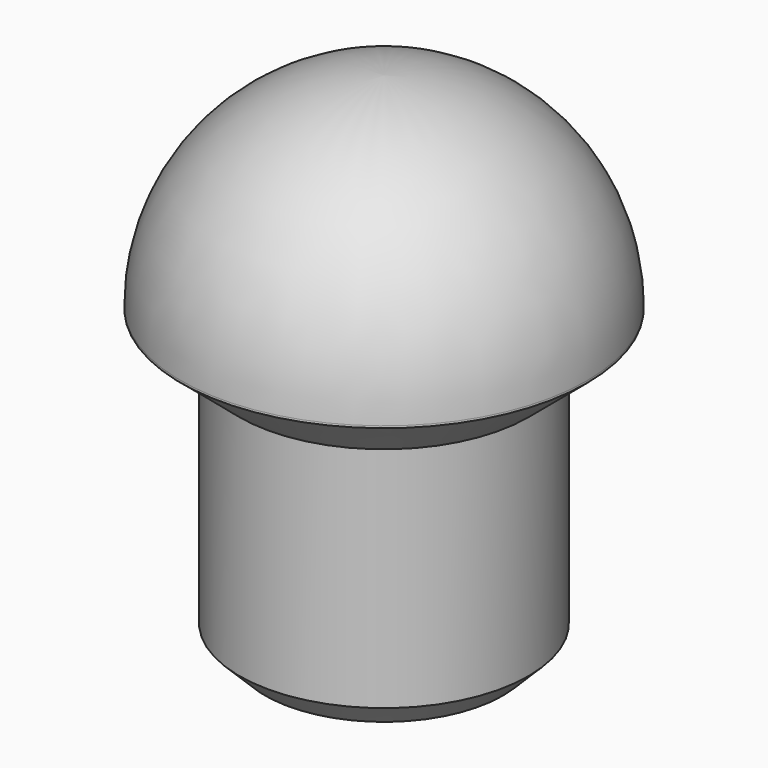
from build123d import *

# Parameters (mm, degrees)
F0_R        = 4
F0_R_2      = 2.85
F1_DEPTH    = 4
F2_DEPTH    = 6
F3_R        = 3.99999
F4_SIZE     = 0.5
F5_S5_R     = 4
F5_T6_DEPTH = 7


# Not quite as in the source:
# - a fillet or chamfer that OpenCascade refuses, or shapes differently, is made with other operations: its cross-section is extruded or revolved along the edge and cut away or added
# - a fillet or chamfer is up to 0.001 mm smaller than in the source, because OpenCascade refuses the exact size


with BuildPart() as f1:
    # F0 (on Top) → F1 (new body)
    with BuildSketch(Plane.XY):
        Circle(F0_R)
        Circle(F0_R_2, mode=Mode.SUBTRACT)
        Circle(F0_R_2)
    extrude(amount=F1_DEPTH)

    # F0 (on Top) → F2 (join)
    with BuildSketch(Plane.XY):
        Circle(F0_R_2)
    extrude(amount=-F2_DEPTH)

    # F3 (radius 4 in the source; OpenCascade refuses exactly that, so slightly less here)
    f3_edges = [f1.edges().sort_by_distance(p)[0] for p in [
        (-4, 0, 4),
    ]]
    fillet(f3_edges, radius=F3_R)

    # F4
    f4_edges = [f1.edges().sort_by_distance(p)[0] for p in [
        (-2.85, 0, -6),
    ]]
    chamfer(f4_edges, length=F4_SIZE)

    # F5: chamfer of 1.2 x 1.0069195574 on 1 edges, made by hand


with BuildPart() as f5_tool2:
    # F5_s3 → F5_t4 (revolve)
    with BuildSketch(Plane.XZ):
        Polygon((2.85, -1.0069195574), (4.05, 0), (2.85, 0), align=None)
    revolve(axis=Axis((0, 0, 0), (0, 0, 1)))

    # F5_s5 → F5_t6 (intersect, symmetric)
    with BuildSketch(Plane.XY.offset(-0.5)):
        Circle(F5_S5_R)
    extrude(amount=F5_T6_DEPTH, both=True, mode=Mode.INTERSECT)


with BuildPart() as f1_1:
    add(f1.part)

    # F5_t1: union F5_tool2
    add(f5_tool2.part)


solid = f1_1.part
